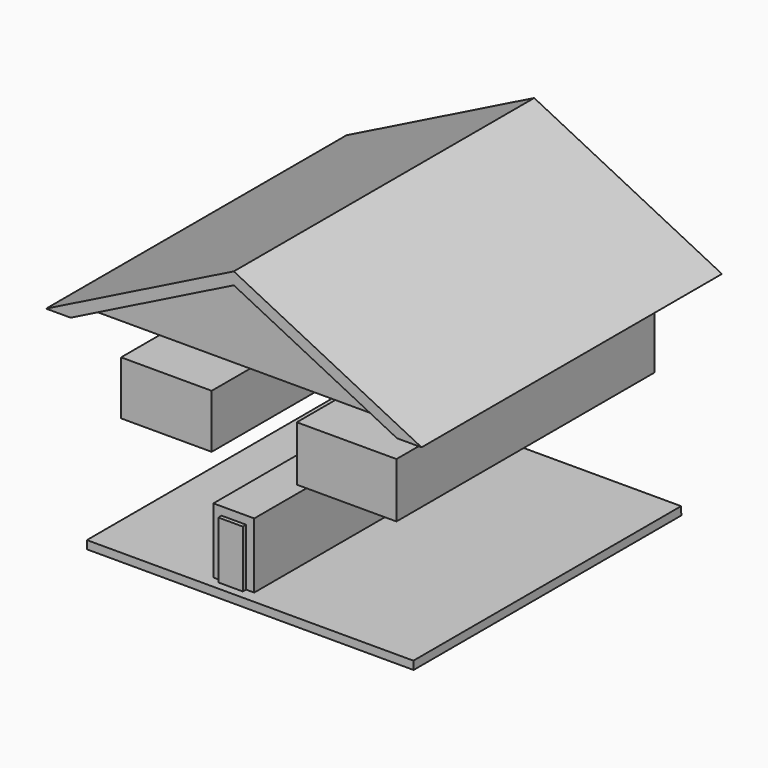
from build123d import *

# Parameters (mm, degrees)
F1_DEPTH = 7010.4
F0_W     = 1828.8
F0_H     = 1524
F2_DEPTH = 6248.4
F3_DEPTH = 6248.4
F4_DEPTH = 6248.4
F0_W_2   = 3382.3656
F0_H_2   = 2006.9420337677
F6_DEPTH = 6019.8
F0_W_3   = 3720.7353115082
F0_H_3   = 2052.0417690277
F7_DEPTH = 6019.8
F0_W_4   = 914.4
F0_H_4   = 2133.6
F8_DEPTH = 5943.6
F9_DEPTH = 5791.2


# Not quite as in the source:
# - the program builds the solid bodies; features that only make, move or delete a surface that nothing else refers to are left out


with BuildPart() as f1:
    # F0 (on Front) → F1 (new body, symmetric)
    with BuildSketch(Plane.XZ):
        Polygon((-7010.4, 0), (-6096, 0), (0, 3048), (0, 3505.2), align=None)
        Polygon((0, 3048), (6096, 0), (7010.4, 0), (0, 3505.2), align=None)
    extrude(amount=F1_DEPTH, both=True)

    # F0 (on Front) → F2 (join, symmetric)
    with BuildSketch(Plane.XZ):
        Polygon((-6096, 0), (0, 0), (6096, 0), (0, 3048), align=None)
        with Locations((-26.6336387634, 1481.3042635918)):
            Rectangle(F0_W, F0_H, mode=Mode.SUBTRACT)
    extrude(amount=F2_DEPTH, both=True)

    # F0 (on Front) → F3 (join, symmetric)
    with BuildSketch(Plane.XZ):
        with Locations((-26.6336387634, 1481.3042635918)):
            Rectangle(F0_W, F0_H)
    extrude(amount=F3_DEPTH, both=True)


with BuildPart() as f4:
    # F0 (on Front) → F4 (new body, symmetric)
    with BuildSketch(Plane.XZ):
        Polygon((-1737.3600006104, -7620), (-6096, -7620), (-6096, -7924.8), (6103.4693717957, -7924.8), (6096, -7620), (-213.3600006104, -7620), (-518.1600006104, -7620), (-1432.5600006104, -7620), align=None)
    extrude(amount=F4_DEPTH, both=True)

    # F0 (on Front) → F8 (join, symmetric)
    with BuildSketch(Plane.XZ):
        with Locations((-975.3600006104, -6553.2)):
            Rectangle(F0_W_4, F0_H_4)
    extrude(amount=F8_DEPTH, both=True)

    # F0 (on Front) → F9 (join, symmetric)
    with BuildSketch(Plane.XZ):
        Polygon((-1737.3600006104, -5181.6), (-1737.3600006104, -7620), (-1432.5600006104, -7620), (-1432.5600006104, -5486.4), (-518.1600006104, -5486.4), (-518.1600006104, -7620), (-213.3600006104, -7620), (-213.3600006104, -5181.6), align=None)
    extrude(amount=F9_DEPTH, both=True)


with BuildPart() as f6:
    # F0 (on Front) → F6 (new body, symmetric)
    with BuildSketch(Plane.XZ):
        with Locations((-3310.5129081657, -2354.0180921555)):
            Rectangle(F0_W_2, F0_H_2)
    extrude(amount=F6_DEPTH, both=True)


with BuildPart() as f7:
    # F0 (on Front) → F7 (new body, symmetric)
    with BuildSketch(Plane.XZ):
        with Locations((3420.6959448952, -2376.5679597855)):
            Rectangle(F0_W_3, F0_H_3)
    extrude(amount=F7_DEPTH, both=True)


solid = Compound([f1.part, f4.part, f6.part, f7.part])
